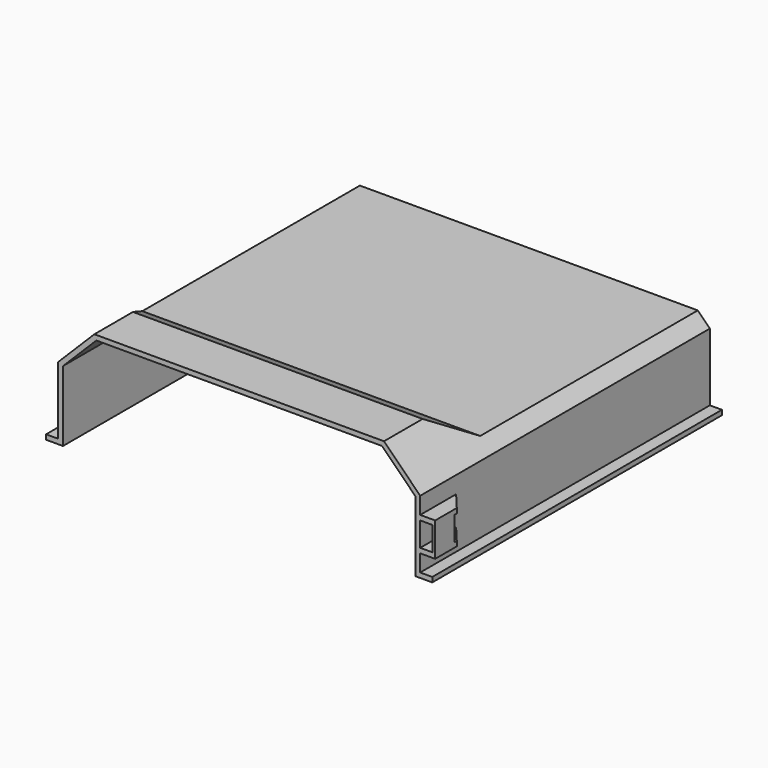
from build123d import *

# Parameters (mm, degrees)
F0_W        = 150
F0_H        = 45
F1_DEPTH    = 150
F2_W        = 5
F2_H        = 150
F3_DEPTH    = 2
F5_DEPTH    = 150
F6_SIZE     = 15
F7_T        = 2
F7_T3_DEPTH = 154
F7_T5_DEPTH = 144
F8_R        = 12.5
F9_DEPTH    = 25
F11_DEPTH   = 10
F13_DEPTH   = 14
F14_W       = 5
F14_H       = 10
F15_DEPTH   = 25
F16_W       = 1.2
F16_H       = 10
F16_W_2     = 1.4301043111
F17_DEPTH   = 6.2


# Not quite as in the source:
# - a shell that OpenCascade refuses in one call is made with other operations: the cavity is built on its own and cut out


with BuildPart() as f1:
    # F0 (on Front) → F1 (new body)
    with BuildSketch(Plane.XZ):
        with Locations((75, 22.5)):
            Rectangle(F0_W, F0_H)
    extrude(amount=F1_DEPTH)

    # F2 (on face) → F3 (join)
    with BuildSketch(Plane(origin=(0, 0, 0), x_dir=(1, 0, 0), z_dir=(0, 0, -1))):
        with Locations((152.5, 75)):
            Rectangle(F2_W, F2_H)
        with Locations((-2.5, 75)):
            Rectangle(F2_W, F2_H)
    extrude(amount=-F3_DEPTH)

    # F4 (on face) → F5 (cut, through all)
    with BuildSketch(Plane.YZ.offset(150)):
        Polygon((0, 35), (0, 45), (-130, 45), (-112.6794919243, 35), align=None)
    extrude(amount=-F5_DEPTH, mode=Mode.SUBTRACT)

    # F6
    f6_edges = [f1.edges().sort_by_distance(p)[0] for p in [
        (0, -140, 45),
        (150, -140, 45),
    ]]
    chamfer(f6_edges, length=F6_SIZE)

    # F7: shell of thickness 2, made by hand


with BuildPart() as f7_core1:
    # F7_t2: copy of F1
    add(f1.part)

    # the walls: a layer under each face that stays
    f7_faces = [f7_core1.faces().sort_by_distance(p)[0] for p in [
        (0, -75, 16),
        (75, 0, 17.5),
        (2.5, -25, 32.5),
        (-2.5, -75, 2),
        (75, -56.3397459622, 35),
        (147.5, -25, 32.5),
        (150, -75, 16),
        (152.5, -75, 2),
        (155, -75, 1),
        (-5, -75, 1),
        (75, -121.3397459622, 40),
        (75, -140, 45),
    ]]
    thicken(f7_faces, amount=-F7_T, mode=Mode.SUBTRACT)

    # F7_s4 → F7_t3 (cut)
    with BuildSketch(Plane.XZ.offset(-2)):
        Polygon((-0.02, 2.02), (2, 2), (2, 0), (0, 0), align=None)
        Polygon((150.02, 2.02), (148, 2), (148, 0), (150, 0), align=None)
    extrude(amount=F7_T3_DEPTH, mode=Mode.SUBTRACT)

    # F7_s6 → F7_t5 (cut)
    with BuildSketch(Plane.YZ.offset(3)):
        Polygon((-112.6694919243, 35.0373205081), (-112.6794919243, 33), (-113.2153903092, 33), (-113.6794919243, 33.2679491924), align=None)
    extrude(amount=F7_T5_DEPTH, mode=Mode.SUBTRACT)


with BuildPart() as f1_1:
    add(f1.part)

    # what is left inside the walls is the cavity
    f7_cavity = [f7_core1.part.solids().sort_by_distance(p)[0] for p in [
        (75, -100.666667, 0.02),
    ]]
    add(f7_cavity, mode=Mode.SUBTRACT)

    # F8 (on face) → F9 (cut)
    with BuildSketch(Plane(origin=(0, 0, 0), x_dir=(-1, 0, 0), z_dir=(0, 1, 0))):
        with Locations((-112.5, 16)):
            Circle(F8_R)
        with Locations((-75, 16)):
            Circle(F8_R)
        with Locations((-37.5, 16)):
            Circle(F8_R)
    extrude(amount=-F9_DEPTH, mode=Mode.SUBTRACT)

    # F10 (on face) → F11 (join)
    with BuildSketch(Plane.XZ.offset(150)):
        Polygon((156.2, 9), (156.2, 23), (150, 23), (150, 21), (155, 21), (155, 11), (150, 11), (150, 9), align=None)
    extrude(amount=-F11_DEPTH)

    # F12 (on face) → F13 (join, through all)
    with BuildSketch(Plane.XY.offset(23)):
        Polygon((150, -140), (156.2, -140), (156.2, -138.8), (150, -131.4111277259), align=None)
    extrude(amount=-F13_DEPTH)

    # F14 (on face) → F15 (cut)
    with BuildSketch(Plane.XZ.offset(150)):
        with Locations((152.5, 16)):
            Rectangle(F14_W, F14_H)
    extrude(amount=-F15_DEPTH, mode=Mode.SUBTRACT)

    # F16 (on face) → F17 (cut, through all)
    with BuildSketch(Plane.YZ.offset(156.2)):
        with Locations((-139.4, 16)):
            Rectangle(F16_W, F16_H)
        with Locations((-138.0849478444, 16)):
            Rectangle(F16_W_2, F16_H)
    extrude(amount=-F17_DEPTH, mode=Mode.SUBTRACT)


solid = f1_1.part
